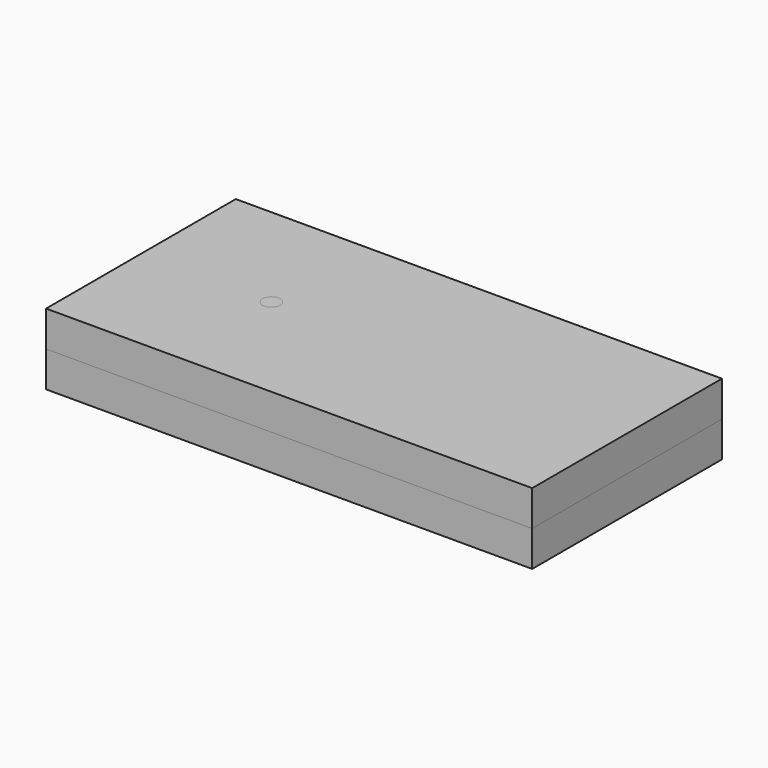
from build123d import *

# Parameters (mm, degrees)
F0_W          = 2000
F0_H          = 1000
F1_DEPTH      = 125
F2_W          = 4100
F2_H          = 2000
F3_DEPTH      = 300
F4_DEPTH      = 300
F6_DEPTH      = 1000
F7_R          = 75
F8_DEPTH      = 300
F8_DEPTH_BACK = 150


with BuildPart() as f1:
    # F0 (on Top) → F1 (new body, symmetric)
    with BuildSketch(Plane.XY):
        Rectangle(F0_W, F0_H)
    extrude(amount=F1_DEPTH, both=True)

    # F5 (on face) → F6 (cut, through all)
    with BuildSketch(Plane.XZ.offset(500)):
        Polygon((-329.8588991165, -125), (-1000, 156.1994105577), (-1000, -125), align=None)
    extrude(amount=-F6_DEPTH, mode=Mode.SUBTRACT)


with BuildPart() as f3:
    # F2 (on Top) → F3 (new body)
    with BuildSketch(Plane.XY):
        with Locations((950, 0)):
            Rectangle(F2_W, F2_H)
    extrude(amount=F3_DEPTH)


with BuildPart() as f4:
    # F2 (on Top) → F4 (new body)
    with BuildSketch(Plane.XY):
        with Locations((950, 0)):
            Rectangle(F2_W, F2_H)
    extrude(amount=-F4_DEPTH)


with BuildPart() as f8:
    # F7 (on Top) → F8 (new body, two sides)
    with BuildSketch(Plane.XY) as f8_sk:
        Circle(F7_R)
    extrude(amount=F8_DEPTH)
    extrude(f8_sk.sketch, amount=-F8_DEPTH_BACK)


solid = Compound([f1.part, f3.part, f4.part, f8.part])
